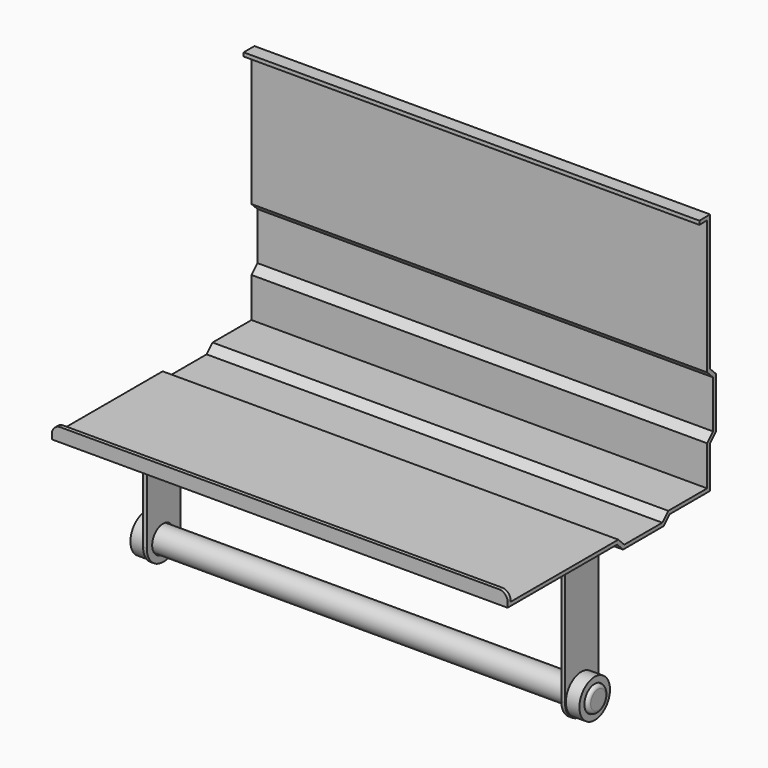
from build123d import *

# Parameters (mm, degrees)
F0_W           = 2.200000473
F0_H           = 2.2
F0_W_2         = 5.799999054
F0_W_3         = 2.2
F0_H_2         = 5.8
F1_DEPTH       = 270
F3_W           = 25
F3_H           = 2.2
F4_DEPTH       = 125
F4_DEPTH_BACK  = 125
F5_W           = 2.2
F5_H           = 25
F6_DEPTH       = 85
F7_R           = 12
F8_R           = 8
F9_DEPTH       = 260.001
F10_R          = 5
F11_R          = 7.5
F12_DEPTH      = 135
F12_DEPTH_BACK = 135
F13_R          = 2
F14_R          = 11.3327676894
F14_R_2        = 7.6443567425
F15_DEPTH      = 8


# Not quite as in the source:
# - ends of sketch curves that miss each other by under 0.0002 mm in the source are joined


with BuildPart() as f1:
    # F0 (on Right) → F1 (new body)
    with BuildSketch(Plane.YZ):
        Polygon((148.3178712445, 90.6965444131), (148.3178712445, 120.6965444131), (143.9178712445, 125.0965444131), (143.9178712445, 195.6965444131), (143.9178716134, 203.4965444131), (141.7178712445, 203.4965444131), (141.7178712445, 124.1852745758), (146.1178712445, 119.7852745758), (146.1178712445, 91.6078142503), (141.7178712445, 87.2078142503), (141.7178712445, 63.6965476274), (143.9178712445, 63.6965476274), (143.9178712445, 86.2965444131), align=None)
        Polygon((143.9178712445, 61.4965476274), (143.9178712445, 63.6965476274), (141.7178712445, 63.6965476274), (112.89533157, 63.6965476274), (108.49533157, 59.2965476274), (80.3178712445, 59.2965476274), (75.9178712445, 63.6965476274), (-3.8821287555, 63.6965476274), (-3.8821287555, 61.4965476274), (75.0066014072, 61.4965476274), (79.4066014072, 57.0965476274), (109.4066014072, 57.0965476274), (113.8066014072, 61.4965476274), align=None)
        with Locations((142.817871481, 204.5965444131)):
            Rectangle(F0_W, F0_H)
        with Locations((138.8178717175, 204.5965444131)):
            Rectangle(F0_W_2, F0_H)
        with Locations((-4.9821287555, 66.5965476274)):
            Rectangle(F0_W_3, F0_H_2)
        with Locations((-4.9821287555, 62.5965476274)):
            Rectangle(F0_W_3, F0_H)
    extrude(amount=F1_DEPTH)

    # F10
    f10_edges = [f1.edges().sort_by_distance(p)[0] for p in [
        (270, -4.982129, 69.496548),
        (0, -4.982129, 69.496548),
    ]]
    fillet(f10_edges, radius=F10_R)


with BuildPart() as f4:
    # F3 (on offset) → F4 (new body, two sides)
    with BuildSketch(Plane(origin=(135, 0, 0), x_dir=(0, -1, 0), z_dir=(-1, 0, 0))) as f4_sk:
        with Locations((-61.4178712445, 60.3965476274)):
            Rectangle(F3_W, F3_H)
    extrude(amount=F4_DEPTH)
    extrude(f4_sk.sketch, amount=-F4_DEPTH_BACK)

    # F5 (on face) → F6 (join)
    with BuildSketch(Plane(origin=(0, 0, 59.2965476274), x_dir=(1, 0, 0), z_dir=(0, 0, -1))):
        with Locations((11.1, -61.4178712445)):
            Rectangle(F5_W, F5_H)
        with Locations((258.9, -61.4178712445)):
            Rectangle(F5_W, F5_H)
    extrude(amount=F6_DEPTH)

    # F7
    f7_edges = [f4.edges().sort_by_distance(p)[0] for p in [
        (258.9, 48.917871, -25.703452),
        (258.9, 73.917871, -25.703452),
        (11.1, 48.917871, -25.703452),
        (11.1, 73.917871, -25.703452),
    ]]
    fillet(f7_edges, radius=F7_R)

    # F8 (on face) → F9 (cut, through all)
    with BuildSketch(Plane.YZ.offset(260)):
        with Locations((60.9178712445, -13.7034523726)):
            Circle(F8_R)
    extrude(amount=-F9_DEPTH, mode=Mode.SUBTRACT)

    # F14 (on face) → F15 (join)
    with BuildSketch(Plane.YZ.offset(260)):
        with Locations((60.9178712445, -13.7034523726)):
            Circle(F14_R)
        with Locations((60.9178712445, -13.7034523726)):
            Circle(F14_R_2, mode=Mode.SUBTRACT)
    extrude(amount=F15_DEPTH)

    # F16: F4 across plane


with BuildPart() as f12:
    # F11 (on offset) → F12 (new body, two sides)
    with BuildSketch(Plane(origin=(135, 0, 0), x_dir=(0, -1, 0), z_dir=(-1, 0, 0))) as f12_sk:
        with Locations((-60.9178712445, -13.7034523726)):
            Circle(F11_R)
    extrude(amount=F12_DEPTH)
    extrude(f12_sk.sketch, amount=-F12_DEPTH_BACK)

    # F13
    f13_edges = [f12.edges().sort_by_distance(p)[0] for p in [
        (270, 68.417871, -13.703452),
        (0, 68.417871, -13.703452),
    ]]
    fillet(f13_edges, radius=F13_R)


with BuildPart() as f4_1:
    add(f4.part)
    add(f4.part.mirror(Plane(origin=(135, 104.2623457429, 98.2578018151), x_dir=(0, 1, 0), z_dir=(-1, 0, 0))))


solid = Compound([f1.part, f12.part, f4_1.part])
